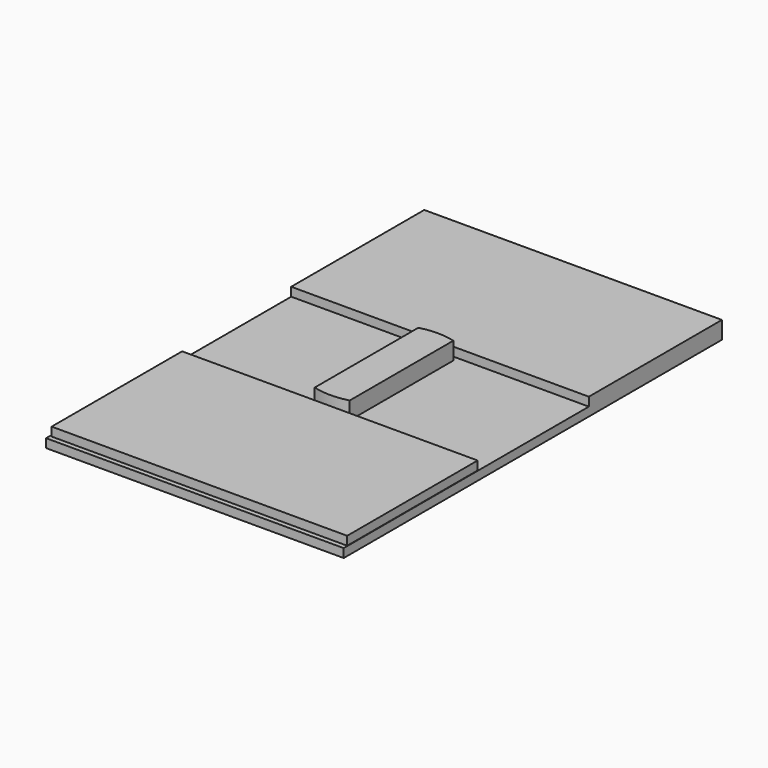
from build123d import *

# Parameters (mm, degrees)
F0_W      = 53.975
F0_H      = 85.725
F1_DEPTH  = 1.5875
F3_W      = 53.5911135375
F3_H      = 29.5717269182
F4_DEPTH  = 1.5875
F2_W      = 53.975
F2_H      = 30.1625
F5_DEPTH  = 1.5875
F9_DEPTH  = 1.5875
F10_DEPTH = 1.5875


# Not quite as in the source:
# - the program builds the solid bodies; features that only make, move or delete a surface that nothing else refers to are left out


with BuildPart() as f1:
    # F0 (on Top) → F1 (new body)
    with BuildSketch(Plane.XY):
        Rectangle(F0_W, F0_H)
    extrude(amount=F1_DEPTH)

    # F3 (on face) → F4 (join)
    with BuildSketch(Plane.XY.offset(1.5875)):
        with Locations((0.1150835305, -27.1980315447)):
            Rectangle(F3_W, F3_H)
    extrude(amount=F4_DEPTH)

    # F2 (on face) → F5 (join)
    with BuildSketch(Plane.XY.offset(1.5875)):
        with Locations((0, 27.78125)):
            Rectangle(F2_W, F2_H)
    extrude(amount=F5_DEPTH)

    # F8 (on face) → F9 (join)
    with BuildSketch(Plane.XY.offset(1.5875)):
        with BuildLine():
            ThreePointArc((-3.175, -11.7439402944), (0, -12.1655562404), (3.175, -11.7439402944))
            Line((3.175, -11.7439402944), (3.175, 11.7439402944))
            ThreePointArc((3.175, 11.7439402944), (0, 12.1655562404), (-3.175, 11.7439402944))
            Line((-3.175, 11.7439402944), (-3.175, -11.7439402944))
        make_face()
    extrude(amount=F9_DEPTH)

    # F10 (add): a face of the model
    f10_faces = [f1.faces().sort_by_distance(p)[0] for p in [
        (0, 0, 3.175),
    ]]
    extrude(f10_faces, amount=F10_DEPTH)


solid = f1.part
